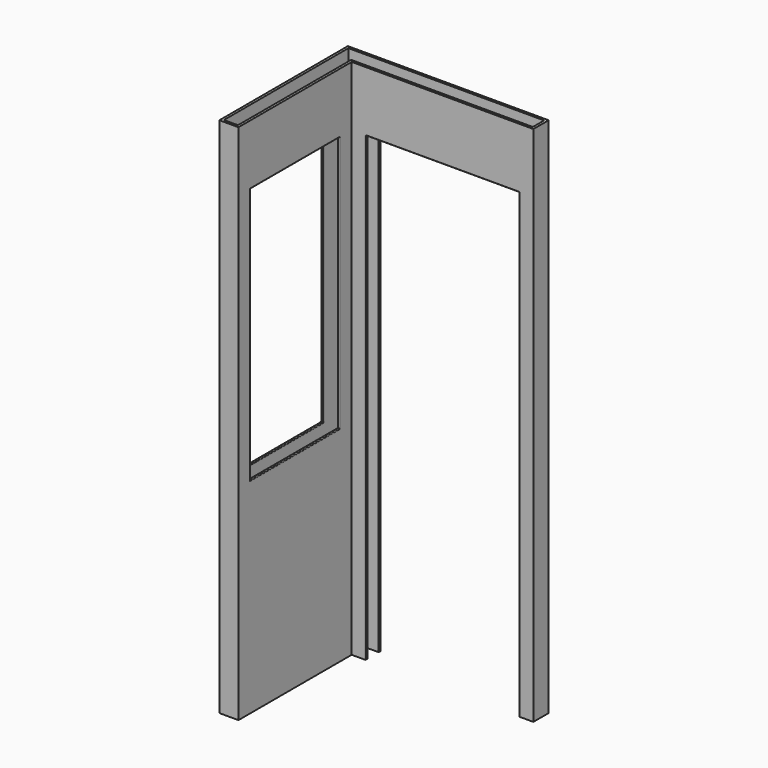
from build123d import *

# Parameters (mm, degrees)
F1_DEPTH = 2600
F2_W     = 560
F2_H     = 1279.0293264389
F3_DEPTH = 95.001
F4_W     = 765
F4_H     = 2300
F5_DEPTH = 95.001
F6_R     = 3


with BuildPart() as f1:
    # F0 (on Top) → F1 (new body)
    with BuildSketch(Plane.XY):
        Polygon((-271.6449069816, 555.1264761336), (-271.6449069816, -244.8735238664), (-176.6449069816, -244.8735238664), (-176.6449069816, 460.1264761336), (728.3550930184, 460.1264761336), (728.3550930184, 555.1264761336), align=None)
        Polygon((-259.1449069816, 542.6264761336), (715.8550930184, 542.6264761336), (715.8550930184, 472.6264761336), (-189.1449069816, 472.6264761336), (-189.1449069816, -232.3735238664), (-259.1449069816, -232.3735238664), align=None, mode=Mode.SUBTRACT)
    extrude(amount=F1_DEPTH)

    # F2 (on face) → F3 (cut, through all)
    with BuildSketch(Plane.YZ.offset(-176.6449069816)):
        with Locations((107.6264761336, 1660.4853367805)):
            Rectangle(F2_W, F2_H)
    extrude(amount=-F3_DEPTH, mode=Mode.SUBTRACT)

    # F4 (on face) → F5 (cut, through all)
    with BuildSketch(Plane.XZ.offset(-460.1264761336)):
        with Locations((275.8550930184, 1150)):
            Rectangle(F4_W, F4_H)
    extrude(amount=-F5_DEPTH, mode=Mode.SUBTRACT)

    # F6
    f6_edges = [f1.edges().sort_by_distance(p)[0] for p in [
        (-106.644907, 542.626476, 1150),
        (-106.644907, 548.876476, 0),
        (-106.644907, 555.126476, 1150),
        (-106.644907, 548.876476, 2300),
        (-106.644907, 460.126476, 1150),
        (-106.644907, 466.376476, 0),
        (-106.644907, 472.626476, 1150),
        (-106.644907, 466.376476, 2300),
        (275.855093, 542.626476, 2300),
        (275.855093, 555.126476, 2300),
        (658.355093, 548.876476, 2300),
        (275.855093, 460.126476, 2300),
        (275.855093, 472.626476, 2300),
        (658.355093, 466.376476, 2300),
        (-259.144907, 107.626476, 2300),
        (-265.394907, -172.373524, 2300),
        (-271.644907, 107.626476, 2300),
        (-265.394907, 387.626476, 2300),
        (-176.644907, 107.626476, 2300),
        (-182.894907, -172.373524, 2300),
        (-189.144907, 107.626476, 2300),
        (-182.894907, 387.626476, 2300),
        (-259.144907, 387.626476, 1660.485337),
        (-271.644907, 387.626476, 1660.485337),
        (-265.394907, 387.626476, 1020.970674),
        (-176.644907, 387.626476, 1660.485337),
        (-189.144907, 387.626476, 1660.485337),
        (-182.894907, 387.626476, 1020.970674),
        (-271.644907, -172.373524, 1660.485337),
        (-271.644907, 107.626476, 1020.970674),
        (658.355093, 555.126476, 1150),
        (-259.144907, -172.373524, 1660.485337),
        (-259.144907, 107.626476, 1020.970674),
        (658.355093, 542.626476, 1150),
        (-189.144907, -172.373524, 1660.485337),
        (-189.144907, 107.626476, 1020.970674),
        (658.355093, 472.626476, 1150),
        (658.355093, 460.126476, 1150),
        (-176.644907, 107.626476, 1020.970674),
        (-176.644907, -172.373524, 1660.485337),
    ]]
    fillet(f6_edges, radius=F6_R)


solid = f1.part
